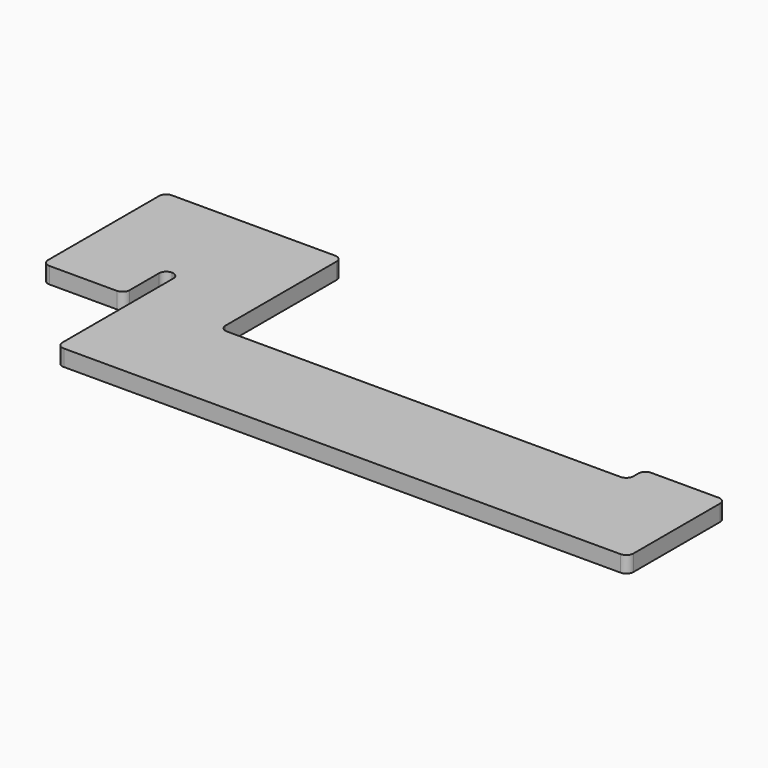
from build123d import *

# Parameters (mm, degrees)
F1_DEPTH = 2.032
F2_R     = 0.88899


# Not quite as in the source:
# - a fillet or chamfer is up to 0.001 mm smaller than in the source, because OpenCascade refuses the exact size


with BuildPart() as f1:
    # F0 (on Top) → F1 (new body)
    with BuildSketch(Plane.XY):
        Polygon((-11.049, 0), (-11.049, -19.05), (-0.889, -19.05), (-0.889, -12.7), (0.889, -12.7), (0.889, -31.75), (72.009, -31.75), (72.009, -16.51), (61.849, -16.51), (61.849, -19.05), (11.049, -19.05), (11.049, 0), align=None)
    extrude(amount=F1_DEPTH)

    # F2 (radius 0.889 in the source; OpenCascade refuses exactly that, so slightly less here)
    f2_edges = [f1.edges().sort_by_distance(p)[0] for p in [
        (-0.889, -12.7, 1.016),
        (0.889, -12.7, 1.016),
        (-0.889, -19.05, 1.016),
        (-11.049, -19.05, 1.016),
        (0.889, -31.75, 1.016),
        (11.049, -19.05, 1.016),
        (72.009, -16.51, 1.016),
        (72.009, -31.75, 1.016),
        (61.849, -16.51, 1.016),
        (61.849, -19.05, 1.016),
        (11.049, 0, 1.016),
        (-11.049, 0, 1.016),
    ]]
    fillet(f2_edges, radius=F2_R)


solid = f1.part
